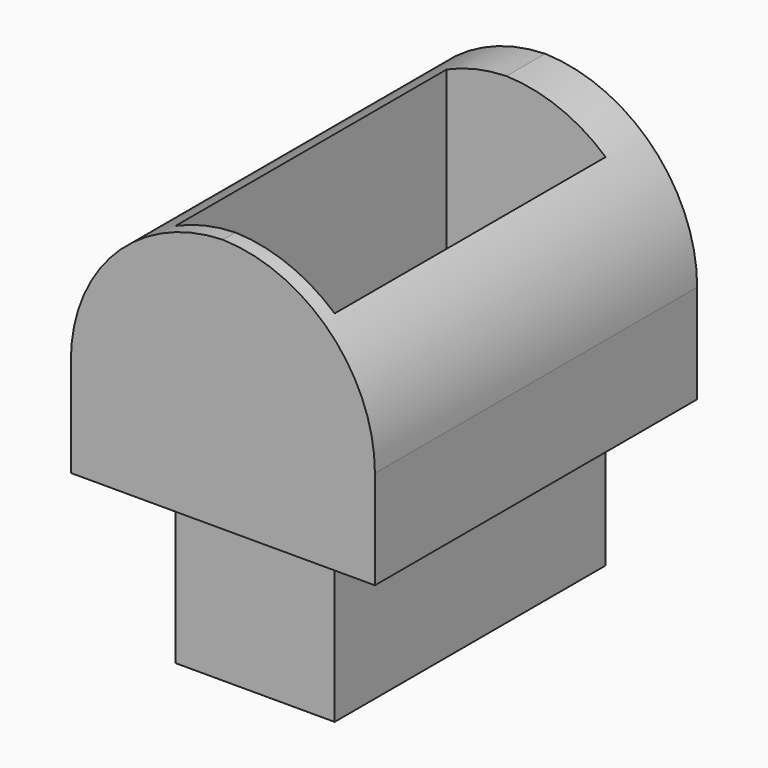
from build123d import *

# Parameters (mm, degrees)
F0_W        = 49.1408258677
F0_H        = 44.438412413
F1_DEPTH    = 104.648
F2_W        = 93.9549271504
F2_H        = 124.46
F2_W_2      = 49.1408258677
F2_H_2      = 104.648
F3_DEPTH    = 78.74
F4_T1_DEPTH = 365.76


# Not quite as in the source:
# - a fillet or chamfer that OpenCascade refuses, or shapes differently, is made with other operations: its cross-section is extruded or revolved along the edge and cut away or added


with BuildPart() as f1:
    # F0 (on Front) → F1 (new body)
    with BuildSketch(Plane.XZ):
        with Locations((-113.5842874646, 32.0855602622)):
            Rectangle(F0_W, F0_H)
    extrude(amount=F1_DEPTH)


with BuildPart() as f3:
    # F2 (on face) → F3 (new body)
    with BuildSketch(Plane.XY.offset(54.3047664687)):
        with Locations((-119.6665391326, -47.2755730152)):
            Rectangle(F2_W, F2_H)
        with Locations((-113.5842874646, -52.324)):
            Rectangle(F2_W_2, F2_H_2, mode=Mode.SUBTRACT)
    extrude(amount=F3_DEPTH)

    # F4: fillet of radius 48.26 on 2 edges, made by hand

    # F4_s2 → F4_t1 (cut)
    with BuildSketch(Plane.XZ.offset(-135.6044269848)):
        with BuildLine():
            ThreePointArc((-72.6890755574, 84.7847664687), (-86.8241022974, 118.9097397288), (-120.9490755574, 133.0447664687))
            Line((-120.9490755574, 133.0447664687), (-72.6890755574, 133.0447664687))
            Line((-72.6890755574, 133.0447664687), (-72.6890755574, 84.7847664687))
        make_face()
        with BuildLine():
            ThreePointArc((-166.6440027078, 84.7847664687), (-152.5089759678, 118.9097397288), (-118.3840027078, 133.0447664687))
            Line((-118.3840027078, 133.0447664687), (-166.6440027078, 133.0447664687))
            Line((-166.6440027078, 133.0447664687), (-166.6440027078, 84.7847664687))
        make_face()
    extrude(amount=F4_T1_DEPTH, mode=Mode.SUBTRACT)


solid = Compound([f1.part, f3.part])
